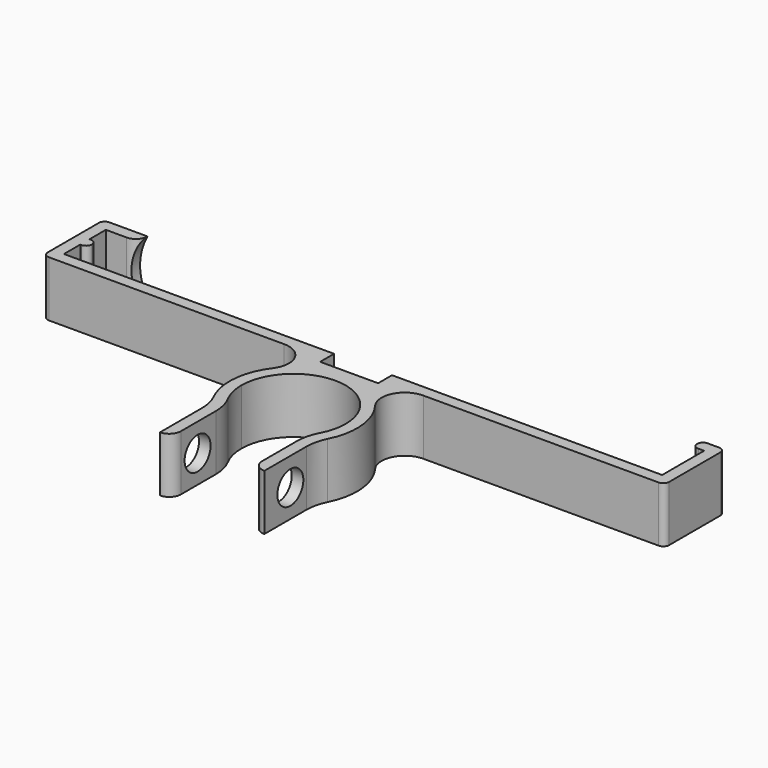
from build123d import *

# Parameters (mm, degrees)
F0_W      = 1.5
F0_H      = 2.5
F1_DEPTH  = 12
F2_R      = 3.5
F3_DEPTH  = 22.5
F4_R      = 10
F5_R      = 2.49999
F6_R      = 1.24999
F7_W      = 12.5
F7_H      = 3.75
F8_DEPTH  = 12
F10_DEPTH = 2.5


# Not quite as in the source:
# - a fillet or chamfer is up to 0.001 mm smaller than in the source, because OpenCascade refuses the exact size


with BuildPart() as f1:
    # F0 (on Top) → F1 (new body)
    with BuildSketch(Plane.XY):
        with BuildLine():
            ThreePointArc((11.25, 0), (10.6066017178, -3.75), (8.75, -7.0710678119))
            Line((8.75, -7.0710678119), (8.75, -10.6066017178))
            ThreePointArc((8.75, -10.6066017178), (10.0907742727, -9.3401699437), (11.25, -7.9056941504))
            Line((11.25, -7.9056941504), (11.25, 0))
        make_face()
        with BuildLine():
            ThreePointArc((-11.25, 0), (0, 11.25), (11.25, 0))
            Line((11.25, 0), (11.25, -7.9056941504))
            ThreePointArc((11.25, -7.9056941504), (13.748354024, 0.2127478073), (11, 8.25))
            ThreePointArc((11, 8.25), (0, 13.75), (-11, 8.25))
            ThreePointArc((-11, 8.25), (-13.748354024, 0.2127478073), (-11.25, -7.9056941504))
            Line((-11.25, -7.9056941504), (-11.25, 0))
        make_face()
        with BuildLine():
            ThreePointArc((11.25, -7.9056941504), (10.0907742727, -9.3401699437), (8.75, -10.6066017178))
            Line((8.75, -10.6066017178), (8.75, -21.9056941504))
            Line((8.75, -21.9056941504), (11.25, -21.9056941504))
            Line((11.25, -21.9056941504), (11.25, -7.9056941504))
        make_face()
        with BuildLine():
            ThreePointArc((-8.75, -7.0710678119), (-10.6066017178, -3.75), (-11.25, 0))
            Line((-11.25, 0), (-11.25, -7.9056941504))
            ThreePointArc((-11.25, -7.9056941504), (-10.0907742727, -9.3401699437), (-8.75, -10.6066017178))
            Line((-8.75, -10.6066017178), (-8.75, -7.0710678119))
        make_face()
        with BuildLine():
            ThreePointArc((-8.75, -10.6066017178), (-10.0907742727, -9.3401699437), (-11.25, -7.9056941504))
            Line((-11.25, -7.9056941504), (-11.25, -21.9056941504))
            Line((-11.25, -21.9056941504), (-8.75, -21.9056941504))
            Line((-8.75, -21.9056941504), (-8.75, -10.6066017178))
        make_face()
        with BuildLine():
            ThreePointArc((-11, 8.25), (0, 13.75), (11, 8.25))
            ThreePointArc((11, 8.25), (10.527864045, 13.4860679775), (15, 16.25))
            Line((15, 16.25), (-15, 16.25))
            ThreePointArc((-15, 16.25), (-10.527864045, 13.4860679775), (-11, 8.25))
        make_face()
        Polygon((-15, 16.25), (15, 16.25), (64.5, 16.25), (64.5, 18.75), (0, 18.75), (-64.5, 18.75), (-64.5, 23.15), (-64.5, 25.65), (-64.5, 30.05), (-67, 30.05), (-67, 16.25), (-64.5, 16.25), align=None)
        Polygon((64.5, 18.75), (64.5, 16.25), (67, 16.25), (67, 30.05), (64.5, 30.05), align=None)
        Polygon((62, 30.05), (64.5, 30.05), (67, 30.05), (67, 32.55), (62, 32.55), align=None)
        Polygon((-67, 32.55), (-67, 30.05), (-64.5, 30.05), (-57.5, 30.05), (-57.5, 32.55), align=None)
        with Locations((-63.75, 24.4)):
            Rectangle(F0_W, F0_H)
    extrude(amount=F1_DEPTH)

    # F2 (on face) → F3 (cut, through all)
    with BuildSketch(Plane(origin=(-11.25, 0, 0), x_dir=(0, -1, 0), z_dir=(-1, 0, 0))):
        with Locations((14.9056941504, 6)):
            Circle(F2_R)
    extrude(amount=-F3_DEPTH, mode=Mode.SUBTRACT)

    # F4
    f4_edges = [f1.edges().sort_by_distance(p)[0] for p in [
        (-8.75, -7.071068, 6),
        (8.75, -7.071068, 6),
        (-11.25, -7.905694, 6),
        (11.25, -7.905694, 6),
    ]]
    fillet(f4_edges, radius=F4_R)

    # F5 (radius 2.5 in the source; OpenCascade refuses exactly that, so slightly less here)
    f5_edges = [f1.edges().sort_by_distance(p)[0] for p in [
        (-57.5, 30.05, 6),
        (-8.75, -21.905694, 6),
        (8.75, -21.905694, 6),
    ]]
    fillet(f5_edges, radius=F5_R)

    # F6 (radius 1.25 in the source; OpenCascade refuses exactly that, so slightly less here)
    f6_edges = [f1.edges().sort_by_distance(p)[0] for p in [
        (-67, 32.55, 6),
        (-67, 16.25, 6),
        (67, 16.25, 6),
        (-63, 23.15, 6),
        (-63, 25.65, 6),
        (62, 32.55, 6),
        (62, 30.05, 6),
        (67, 32.55, 6),
    ]]
    fillet(f6_edges, radius=F6_R)

    # F7 (on face) → F8 (cut, through all)
    with BuildSketch(Plane.XY.offset(12)):
        with Locations((0, 16.875)):
            Rectangle(F7_W, F7_H)
    extrude(amount=-F8_DEPTH, mode=Mode.SUBTRACT)

    # F9 (on face) → F10 (cut, through all)
    with BuildSketch(Plane(origin=(0, 32.55, 0), x_dir=(-1, 0, 0), z_dir=(0, 1, 0))):
        with BuildLine():
            Line((57.5, 12), (57.5, 0))
            ThreePointArc((57.5, 0), (59.1076951546, 6), (57.5, 12))
        make_face()
    extrude(amount=-F10_DEPTH, mode=Mode.SUBTRACT)


solid = f1.part
